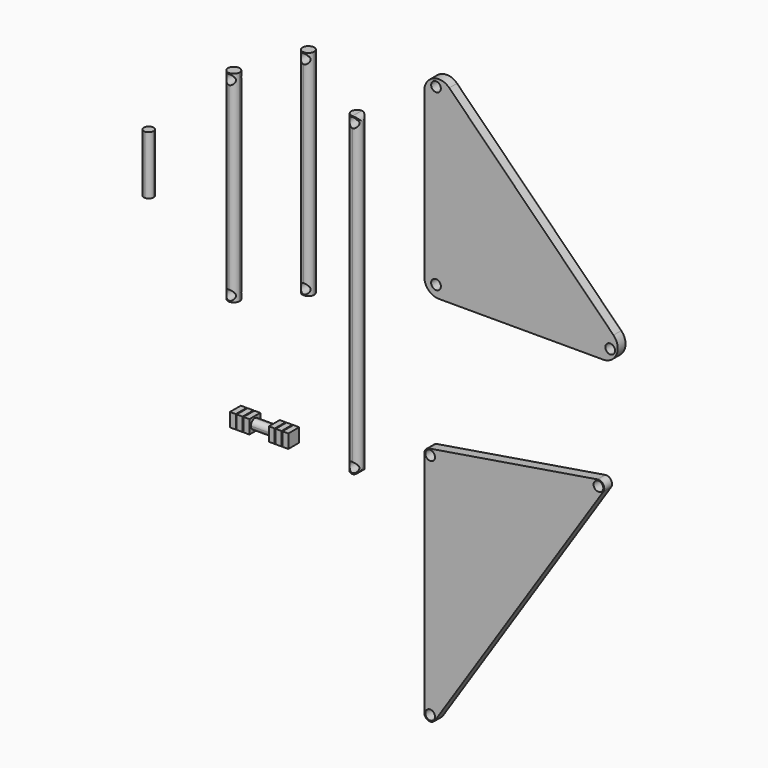
from build123d import *

# Parameters (mm, degrees)
F1_DEPTH       = 12.7
F3_D           = 12.7
F4_R           = 19.05
F5_W           = 15.24
F5_H           = 279.4
F5_R           = 6.35
F6_DEPTH       = 15.24
F7_T1_DEPTH    = 317.5
F8_W           = 15.24
F8_H           = 262.89
F8_R           = 6.35
F9_DEPTH       = 15.24
F10_T1_DEPTH   = 300.99
F11_R          = 6.35
F12_DEPTH      = 12.7
F13_R          = 7.62
F14_W          = 76.2
F14_H          = 12.7
F15_DEPTH      = 12.7
F16_W          = 7.62
F16_H          = 12.7
F17_DEPTH      = 2.54
F17_DEPTH_BACK = 15.24
F19_DEPTH      = 2.54
F19_DEPTH_BACK = 15.24
F20_R          = 6.34999
F21_W          = 12.7
F21_H          = 76.2
F22_DEPTH      = 12.7
F23_R          = 6.34999
F24_W          = 15.24
F24_H          = 411.48
F25_DEPTH      = 15.24
F26_D          = 12.7
F27_T1_DEPTH   = 449.58
F27_T3_DEPTH   = 53.34


# Not quite as in the source:
# - a fillet or chamfer that OpenCascade refuses, or shapes differently, is made with other operations: its cross-section is extruded or revolved along the edge and cut away or added
# - a fillet or chamfer is up to 0.001 mm smaller than in the source, because OpenCascade refuses the exact size


with BuildPart() as f1:
    # F0 (on Front) → F1 (new body)
    with BuildSketch(Plane.XZ):
        Polygon((0, 279.4), (0, 0), (279.4, 0), align=None)
    extrude(amount=F1_DEPTH)

    # F3 (through all)
    with Locations(Plane(origin=(0, 0, 0), x_dir=(-1, 0, 0), z_dir=(0, 1, 0))):
        with Locations((-242.6073853094, 15.24), (-15.24, 15.24), (-15.24, 242.6073853094)):
            Hole(F3_D / 2)

    # F4
    f4_edges = [f1.edges().sort_by_distance(p)[0] for p in [
        (0, -6.35, 0),
        (0, -6.35, 279.4),
        (279.4, -6.35, 0),
    ]]
    fillet(f4_edges, radius=F4_R)


with BuildPart() as f6:
    # F5 (on Front) → F6 (new body)
    with BuildSketch(Plane.XZ):
        with Locations((-155.3884372115, 88.0704151236)):
            Rectangle(F5_W, F5_H)
        with Locations((-155.3884372115, -44.0095848764)):
            Circle(F5_R, mode=Mode.SUBTRACT)
        with Locations((-155.3884372115, 220.1504151236)):
            Circle(F5_R, mode=Mode.SUBTRACT)
    extrude(amount=F6_DEPTH)

    # F7: fillet of radius 7.62 on 4 edges, made by hand

    # F7_s2 → F7_t1 (cut)
    with BuildSketch(Plane.XY.offset(-70.6795848764)):
        with BuildLine():
            ThreePointArc((-163.0084372115, -7.62), (-160.7765908842, -13.0081536726), (-155.3884372115, -15.24))
            Line((-155.3884372115, -15.24), (-163.0084372115, -15.24))
            Line((-163.0084372115, -15.24), (-163.0084372115, -7.62))
        make_face()
        with BuildLine():
            ThreePointArc((-147.7684372115, -7.62), (-150.0002835389, -13.0081536726), (-155.3884372115, -15.24))
            Line((-155.3884372115, -15.24), (-147.7684372115, -15.24))
            Line((-147.7684372115, -15.24), (-147.7684372115, -7.62))
        make_face()
        with BuildLine():
            ThreePointArc((-147.7684372115, -7.62), (-150.0002835389, -2.2318463274), (-155.3884372115, 0))
            Line((-155.3884372115, 0), (-147.7684372115, 0))
            Line((-147.7684372115, 0), (-147.7684372115, -7.62))
        make_face()
        with BuildLine():
            ThreePointArc((-163.0084372115, -7.62), (-160.7765908842, -2.2318463274), (-155.3884372115, 0))
            Line((-155.3884372115, 0), (-163.0084372115, 0))
            Line((-163.0084372115, 0), (-163.0084372115, -7.62))
        make_face()
    extrude(amount=F7_T1_DEPTH, mode=Mode.SUBTRACT)


with BuildPart() as f9:
    # F8 (on Front) → F9 (new body)
    with BuildSketch(Plane.XZ):
        with Locations((-252.7289167047, 40.8442549972)):
            Rectangle(F8_W, F8_H)
        with Locations((-252.7289167047, -82.9807450028)):
            Circle(F8_R, mode=Mode.SUBTRACT)
        with Locations((-252.7289167047, 164.6692549972)):
            Circle(F8_R, mode=Mode.SUBTRACT)
    extrude(amount=F9_DEPTH)

    # F10: fillet of radius 7.62 on 4 edges, made by hand

    # F10_s2 → F10_t1 (cut)
    with BuildSketch(Plane.XY.offset(-109.6507450028)):
        with BuildLine():
            ThreePointArc((-260.3489167047, -7.62), (-258.1170703773, -13.0081536726), (-252.7289167047, -15.24))
            Line((-252.7289167047, -15.24), (-260.3489167047, -15.24))
            Line((-260.3489167047, -15.24), (-260.3489167047, -7.62))
        make_face()
        with BuildLine():
            ThreePointArc((-245.1089167047, -7.62), (-247.340763032, -13.0081536726), (-252.7289167047, -15.24))
            Line((-252.7289167047, -15.24), (-245.1089167047, -15.24))
            Line((-245.1089167047, -15.24), (-245.1089167047, -7.62))
        make_face()
        with BuildLine():
            ThreePointArc((-260.3489167047, -7.62), (-258.1170703773, -2.2318463274), (-252.7289167047, 0))
            Line((-252.7289167047, 0), (-260.3489167047, 0))
            Line((-260.3489167047, 0), (-260.3489167047, -7.62))
        make_face()
        with BuildLine():
            ThreePointArc((-245.1089167047, -7.62), (-247.340763032, -2.2318463274), (-252.7289167047, 0))
            Line((-252.7289167047, 0), (-245.1089167047, 0))
            Line((-245.1089167047, 0), (-245.1089167047, -7.62))
        make_face()
    extrude(amount=F10_T1_DEPTH, mode=Mode.SUBTRACT)


with BuildPart() as f12:
    # F11 (on Front) → F12 (new body)
    with BuildSketch(Plane.XZ):
        Polygon((243.1481603684, -137.2364790053), (0, -177.01180439), (0, -507.21180439), align=None)
        with Locations((7.62, -481.7427504187)):
            Circle(F11_R, mode=Mode.SUBTRACT)
        with Locations((7.62, -183.4865711255)):
            Circle(F11_R, mode=Mode.SUBTRACT)
        with Locations((227.2458065223, -147.5591435684)):
            Circle(F11_R, mode=Mode.SUBTRACT)
    extrude(amount=F12_DEPTH)

    # F13
    f13_edges = [f12.edges().sort_by_distance(p)[0] for p in [
        (243.14816, -6.35, -137.236479),
        (0, -6.35, -507.211804),
        (0, -6.35, -177.011804),
    ]]
    fillet(f13_edges, radius=F13_R)


with BuildPart() as f15:
    # F14 (on Front) → F15 (new body)
    with BuildSketch(Plane.XZ):
        with Locations((-213.5778516531, -225.7402785766)):
            Rectangle(F14_W, F14_H)
    extrude(amount=F15_DEPTH)

    # F16 (on face) → F17 (join, two sides)
    with BuildSketch(Plane.XZ.offset(12.7)) as f17_sk:
        with Locations((-247.8678516531, -225.7402785766)):
            Rectangle(F16_W, F16_H)
        with Locations((-238.9778516531, -225.7402785766)):
            Rectangle(F16_W, F16_H)
        with Locations((-230.0878516531, -225.7402785766)):
            Rectangle(F16_W, F16_H)
        with Locations((-197.0678516531, -225.7402785766)):
            Rectangle(F16_W, F16_H)
        with Locations((-188.1778516531, -225.7402785766)):
            Rectangle(F16_W, F16_H)
        with Locations((-179.2878516531, -225.7402785766)):
            Rectangle(F16_W, F16_H)
    extrude(amount=F17_DEPTH)
    extrude(f17_sk.sketch, amount=-F17_DEPTH_BACK)

    # F18 (on face) → F19 (join, two sides)
    with BuildSketch(Plane.XY.offset(-219.3902785766)) as f19_sk:
        Polygon((-244.0578516531, -12.7), (-244.0578516531, 0), (-244.0578516531, 2.54), (-251.6778516531, 2.54), (-251.6778516531, -15.24), (-244.0578516531, -15.24), align=None)
        Polygon((-242.7878516531, 2.54), (-242.7878516531, 0), (-242.7878516531, -12.7), (-242.7878516531, -15.24), (-235.1678516531, -15.24), (-235.1678516531, -12.7), (-235.1678516531, 0), (-235.1678516531, 2.54), align=None)
        Polygon((-233.8978516531, 2.54), (-233.8978516531, 0), (-233.8978516531, -12.7), (-233.8978516531, -15.24), (-226.2778516531, -15.24), (-226.2778516531, -12.7), (-226.2778516531, 0), (-226.2778516531, 2.54), align=None)
        Polygon((-200.8778516531, 2.54), (-200.8778516531, 0), (-200.8778516531, -12.7), (-200.8778516531, -15.24), (-193.2578516531, -15.24), (-193.2578516531, -12.7), (-193.2578516531, 0), (-193.2578516531, 2.54), align=None)
        Polygon((-191.9878516531, 2.54), (-191.9878516531, 0), (-191.9878516531, -12.7), (-191.9878516531, -15.24), (-184.3678516531, -15.24), (-184.3678516531, -12.7), (-184.3678516531, 0), (-184.3678516531, 2.54), align=None)
        Polygon((-183.0978516531, 2.54), (-183.0978516531, 0), (-183.0978516531, -12.7), (-183.0978516531, -15.24), (-175.4778516531, -15.24), (-175.4778516531, 2.54), align=None)
    extrude(amount=F19_DEPTH)
    extrude(f19_sk.sketch, amount=-F19_DEPTH_BACK)

    # F20 (radius 6.35 in the source; OpenCascade refuses exactly that, so slightly less here)
    f20_edges = [f15.edges().sort_by_distance(p)[0] for p in [
        (-213.577852, -12.7, -219.390279),
        (-213.577852, -12.7, -232.090279),
        (-213.577852, 0, -232.090279),
        (-213.577852, 0, -219.390279),
    ]]
    fillet(f20_edges, radius=F20_R)


with BuildPart() as f22:
    # F21 (on Front) → F22 (new body)
    with BuildSketch(Plane.XZ):
        with Locations((-364.8103475571, 29.3068300472)):
            Rectangle(F21_W, F21_H)
    extrude(amount=F22_DEPTH)

    # F23 (radius 6.35 in the source; OpenCascade refuses exactly that, so slightly less here)
    f23_edges = [f22.edges().sort_by_distance(p)[0] for p in [
        (-371.160348, -12.7, 29.30683),
        (-358.460348, -12.7, 29.30683),
        (-358.460348, 0, 29.30683),
        (-371.160348, 0, 29.30683),
    ]]
    fillet(f23_edges, radius=F23_R)


with BuildPart() as f25:
    # F24 (on Front) → F25 (new body)
    with BuildSketch(Plane.XZ):
        with Locations((-91.7072184384, -30.5626919081)):
            Rectangle(F24_W, F24_H)
    extrude(amount=F25_DEPTH)

    # F26 (through all)
    with Locations(Plane(origin=(0, 0, 0), x_dir=(1, 0, 0), z_dir=(0, 1, 0))):
        with Locations((-91.7072184384, -167.5573080919), (-91.7072184384, 228.6826919081)):
            Hole(F26_D / 2)

    # F27: fillet of radius 7.62 on 6 edges, made by hand

    # F27_s2 → F27_t1 (cut)
    with BuildSketch(Plane.XY.offset(-255.3526919081)):
        with BuildLine():
            ThreePointArc((-91.7072184384, 0), (-97.095372111, -2.2318463274), (-99.3272184384, -7.62))
            Line((-99.3272184384, -7.62), (-99.3272184384, 0))
            Line((-99.3272184384, 0), (-91.7072184384, 0))
        make_face()
        with BuildLine():
            ThreePointArc((-91.7072184384, -15.24), (-97.095372111, -13.0081536726), (-99.3272184384, -7.62))
            Line((-99.3272184384, -7.62), (-99.3272184384, -15.24))
            Line((-99.3272184384, -15.24), (-91.7072184384, -15.24))
        make_face()
        with BuildLine():
            ThreePointArc((-84.0872184384, -7.62), (-86.3190647657, -13.0081536726), (-91.7072184384, -15.24))
            Line((-91.7072184384, -15.24), (-84.0872184384, -15.24))
            Line((-84.0872184384, -15.24), (-84.0872184384, -7.62))
        make_face()
        with BuildLine():
            ThreePointArc((-84.0872184384, -7.62), (-86.3190647657, -2.2318463274), (-91.7072184384, 0))
            Line((-91.7072184384, 0), (-84.0872184384, 0))
            Line((-84.0872184384, 0), (-84.0872184384, -7.62))
        make_face()
    extrude(amount=F27_T1_DEPTH, mode=Mode.SUBTRACT)

    # F27_s4 → F27_t3 (cut)
    with BuildSketch(Plane.XZ.offset(-19.05)):
        with BuildLine():
            ThreePointArc((-84.0872184384, -228.6826919081), (-86.3190647657, -234.0708455807), (-91.7072184384, -236.3026919081))
            Line((-91.7072184384, -236.3026919081), (-84.0872184384, -236.3026919081))
            Line((-84.0872184384, -236.3026919081), (-84.0872184384, -228.6826919081))
        make_face()
        with BuildLine():
            ThreePointArc((-84.0872184384, 167.5573080919), (-86.3190647657, 172.9454617646), (-91.7072184384, 175.1773080919))
            Line((-91.7072184384, 175.1773080919), (-84.0872184384, 175.1773080919))
            Line((-84.0872184384, 175.1773080919), (-84.0872184384, 167.5573080919))
        make_face()
    extrude(amount=F27_T3_DEPTH, mode=Mode.SUBTRACT)


solid = Compound([f1.part, f6.part, f9.part, f12.part, f15.part, f22.part, f25.part])
